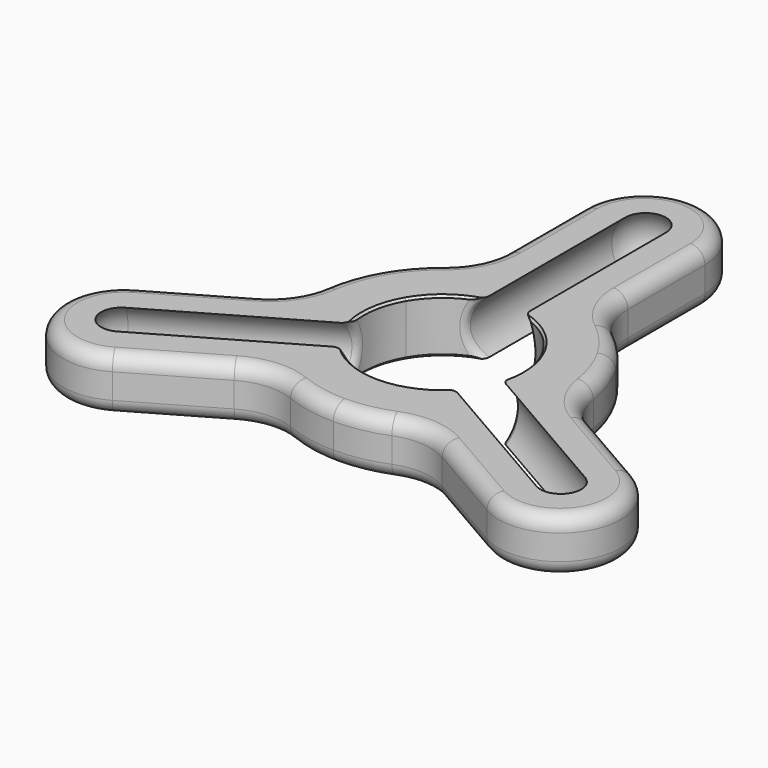
from build123d import *

# Parameters (mm, degrees)
F1_DEPTH      = 3.75
F1_DEPTH_BACK = 3.75
F2_R          = 4.7
F4_DEPTH      = 40
F5_R          = 4.7
F6_R          = 8.5
F8_T2_ANGLE   = 53.1118954737
F8_T4_ANGLE   = 53.1118954737
F8_T6_ANGLE   = 53.1118954737
F8_T8_ANGLE   = 53.1118954737
F9_R          = 1.2
F10_COUNT     = 3
F11_R         = 2


# Not quite as in the source:
# - a fillet or chamfer that OpenCascade refuses, or shapes differently, is made with other operations: its cross-section is extruded or revolved along the edge and cut away or added


with BuildPart() as f1:
    # F0 (on Top) → F1 (new body, two sides)
    with BuildSketch(Plane.XY) as f1_sk:
        with BuildLine():
            ThreePointArc((-9.5262794416, 5.5), (0, 11), (9.5262794416, 5.5))
            Line((9.5262794416, 5.5), (16.4544826719, 9.5))
            ThreePointArc((16.4544826719, 9.5), (13.0275279843, 13.8305283564), (8.5, 16.992645468))
            Line((8.5, 16.992645468), (8.5, 35))
            ThreePointArc((8.5, 35), (0, 43.5), (-8.5, 35))
            Line((-8.5, 35), (-8.5, 16.992645468))
            ThreePointArc((-8.5, 16.992645468), (-13.0275279843, 13.8305283564), (-16.4544826719, 9.5))
            Line((-16.4544826719, 9.5), (-9.5262794416, 5.5))
        make_face()
    extrude(amount=F1_DEPTH)
    extrude(f1_sk.sketch, amount=-F1_DEPTH_BACK)

    # F6
    f6_edges = [f1.edges().sort_by_distance(p)[0] for p in [
        (-8.5, 16.992645, 0),
        (8.5, 16.992645, 0),
    ]]
    fillet(f6_edges, radius=F6_R)


with BuildPart() as f4:
    # F2 (on Front) → F4 (new body)
    with BuildSketch(Plane.XZ):
        Circle(F2_R)
    extrude(amount=-F4_DEPTH)

    # F5
    f5_edges = [f4.edges().sort_by_distance(p)[0] for p in [
        (-4.7, 40, 0),
    ]]
    fillet(f5_edges, radius=F5_R)


with BuildPart() as f1_1:
    add(f1.part)

    # F7: cut F4
    add(f4.part, mode=Mode.SUBTRACT)

    # F8: chamfer of 0.3 on 4 edges, made by hand

    # F8_s1 → F8_t2 (revolve, cut)
    with BuildSketch(Plane(origin=(0, 0, 0), x_dir=(0, 0, 1), z_dir=(-0.438073888, -0.8989389682, 0))):
        Polygon((3.75, 11.3), (3.45, 11), (3.75, 11), align=None)
    revolve(axis=Axis((0, 0, 3.75), (0, 0, -1)), revolution_arc=F8_T2_ANGLE, mode=Mode.SUBTRACT)

    # F8_s3 → F8_t4 (revolve, cut)
    with BuildSketch(Plane(origin=(0, 0, 0), x_dir=(0, 0, 1), z_dir=(-0.438073888, -0.8989389682, 0))):
        Polygon((-3.75, 11.3), (-3.45, 11), (-3.75, 11), align=None)
    revolve(axis=Axis((0, 0, -3.75), (0, 0, -1)), revolution_arc=F8_T4_ANGLE, mode=Mode.SUBTRACT)

    # F8_s5 → F8_t6 (revolve, cut)
    with BuildSketch(Plane(origin=(0, 0, 0), x_dir=(0, 0, 1), z_dir=(-0.9819354297, 0.1892163097, 0))):
        Polygon((-3.75, 11.3), (-3.45, 11), (-3.75, 11), align=None)
    revolve(axis=Axis((0, 0, -3.75), (0, 0, -1)), revolution_arc=F8_T6_ANGLE, mode=Mode.SUBTRACT)

    # F8_s7 → F8_t8 (revolve, cut)
    with BuildSketch(Plane(origin=(0, 0, 0), x_dir=(0, 0, 1), z_dir=(-0.9819354297, 0.1892163097, 0))):
        Polygon((3.75, 11.3), (3.45, 11), (3.75, 11), align=None)
    revolve(axis=Axis((0, 0, 3.75), (0, 0, -1)), revolution_arc=F8_T8_ANGLE, mode=Mode.SUBTRACT)

    # F9
    f9_edges = [f1_1.edges().sort_by_distance(p)[0] for p in [
        (-4.7, 9.945351, 0),
        (4.7, 9.945351, 0),
    ]]
    fillet(f9_edges, radius=F9_R)

    # F10: F1 ×3 about axis
    f10_axis = Axis((0, 0, 12.4659836292), (0, 0, 1))


with BuildPart() as f1_2:
    add(f1_1.part)
    for i in range(1, F10_COUNT):
        add(f1_1.part.rotate(f10_axis, i * 360 / F10_COUNT))

    # F11
    f11_edges = [f1_2.edges().sort_by_distance(p)[0] for p in [
        (-8.5, 28.307983, 3.75),
        (-20.265433, -21.515208, -3.75),
    ]]
    fillet(f11_edges, radius=F11_R)


solid = f1_2.part
